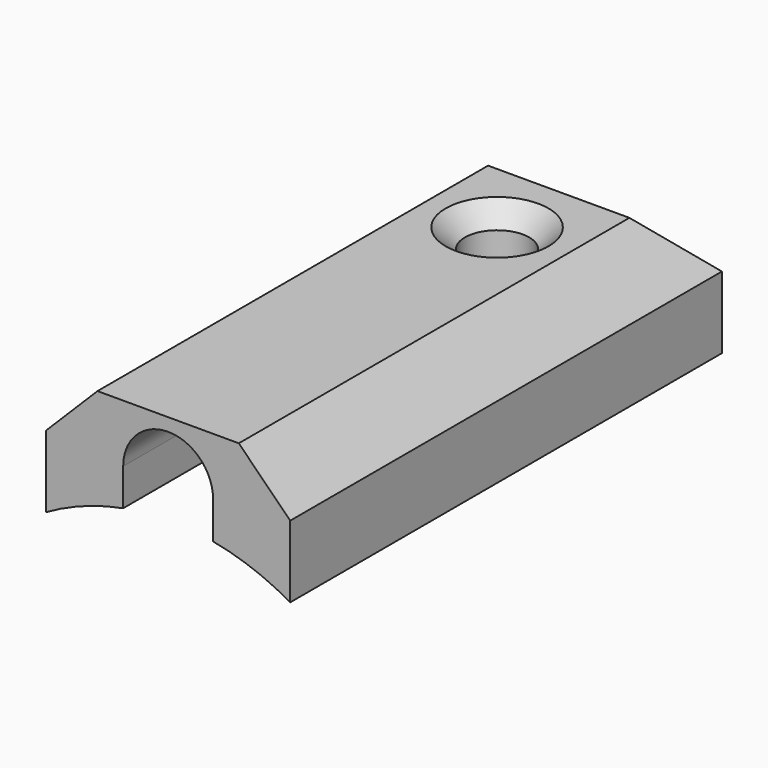
from build123d import *

# Parameters (mm, degrees)
F6_DEPTH        = 21
F7_SIZE         = 2
F8_SIZE         = 2
F12_DEPTH       = 2.5510001
F14_D           = 2.5
F14_CSINK_D     = 4
F14_CSINK_ANGLE = 90


# Not quite as in the source:
# - a feature names something its author has since deleted; it is built from what else it names


with BuildPart() as f6:
    # F5 (on Front) → F6 (new body)
    with BuildSketch(Plane.XZ):
        with BuildLine():
            ThreePointArc((1.75, 9.3374246985), (3.2970633562, 8.9095102685), (4.75, 8.227241336))
            Line((4.75, 8.227241336), (4.75, 13.027241336))
            Line((4.75, 13.027241336), (-4.75, 13.027241336))
            Line((-4.75, 13.027241336), (-4.75, 8.227241336))
            ThreePointArc((-4.75, 8.227241336), (-3.2970633562, 8.9095102685), (-1.75, 9.3374246985))
            Line((-1.75, 9.3374246985), (-1.75, 10.777241336))
            ThreePointArc((-1.75, 10.777241336), (0, 12.527241336), (1.75, 10.777241336))
            Line((1.75, 10.777241336), (1.75, 9.3374246985))
        make_face()
        with BuildLine():
            ThreePointArc((-1.75, 9.3374246985), (0, 9.5), (1.75, 9.3374246985))
            Line((1.75, 9.3374246985), (1.75, 10.777241336))
            ThreePointArc((1.75, 10.777241336), (0, 12.527241336), (-1.75, 10.777241336))
            Line((-1.75, 10.777241336), (-1.75, 9.3374246985))
        make_face()
    extrude(amount=-F6_DEPTH)

    # F7
    f7_edges = [f6.edges().sort_by_distance(p)[0] for p in [
        (-4.75, 10.5, 13.027241),
        (4.75, 10.5, 13.027241),
    ]]
    chamfer(f7_edges, length=F7_SIZE)

    # F8
    f8_edges = [f6.edges().sort_by_distance(p)[0] for p in [
        (0, 21, 13.027241),
    ]]
    chamfer(f8_edges, length=F8_SIZE)

    # F10 (on offset) → F11 (revolve, cut)
    with BuildSketch(Plane.XY.offset(10.777241336)):
        with BuildLine():
            Line((-1.75, 11.75), (-1.75, 0))
            Line((-1.75, 0), (0, 0))
            Line((0, 0), (0, 13.5))
            ThreePointArc((0, 13.5), (-1.2374368671, 12.9874368671), (-1.75, 11.75))
        make_face()
    revolve(axis=Axis((0, 6.75, 10.777241336), (0, 1, 0)), mode=Mode.SUBTRACT)

    # F10 (on offset) → F12 (cut, through all)
    with BuildSketch(Plane.XY.offset(10.777241336)):
        with BuildLine():
            Line((0, 13.5), (0, 0))
            Line((0, 0), (1.75, 0))
            Line((1.75, 0), (1.75, 11.75))
            ThreePointArc((1.75, 11.75), (1.2374368671, 12.9874368671), (0, 13.5))
        make_face()
        with BuildLine():
            Line((-1.75, 11.75), (-1.75, 0))
            Line((-1.75, 0), (0, 0))
            Line((0, 0), (0, 13.5))
            ThreePointArc((0, 13.5), (-1.2374368671, 12.9874368671), (-1.75, 11.75))
        make_face()
    extrude(amount=-F12_DEPTH, mode=Mode.SUBTRACT)

    # F14 (through all)
    with Locations(Plane.XY.offset(13.027241336)):
        with Locations((0, 16)):
            CounterSinkHole(F14_D / 2, F14_CSINK_D / 2, counter_sink_angle=F14_CSINK_ANGLE)


solid = f6.part
